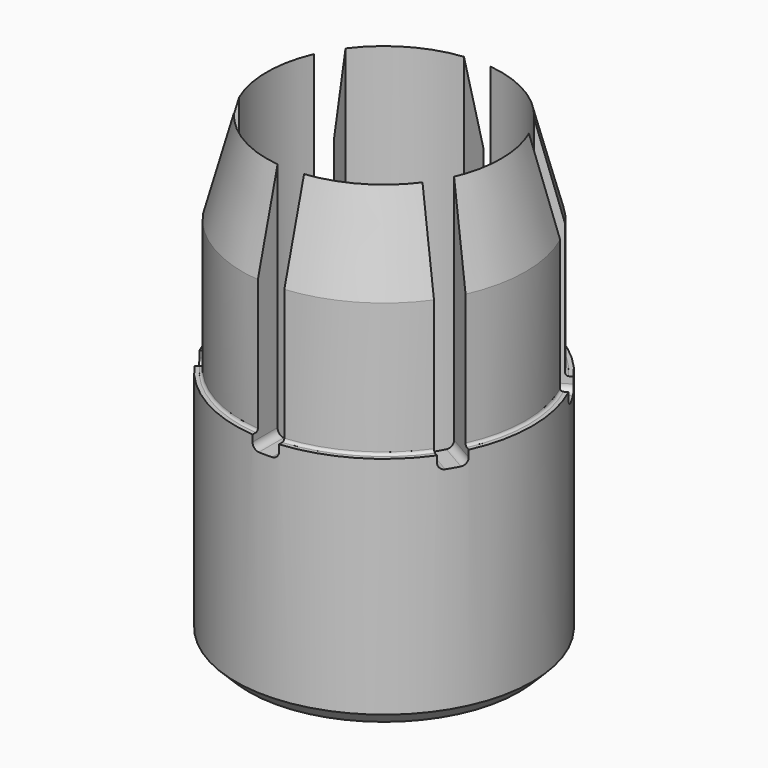
from build123d import *

# Parameters (mm, degrees)
F3_SIZE         = 0.254
F4_W            = 0.508
F4_H            = 3.048
F6_DEPTH        = 4.572
F6_COPIES_COUNT = 6
F7_R            = 0.127
F8_R            = 0.0508


# Not quite as in the source:
# - a pattern or mirror of a feature is missing from the dataset's text; its kind, count and spacing are read off the source's solid


with BuildPart() as f1:
    # F0 (on Front) → F1 (revolve)
    with BuildSketch(Plane.XZ):
        with BuildLine():
            Line((2.2098, 0), (2.8448, 0))
            Line((2.8448, 0), (2.8448, 4.572))
            Line((2.8448, 4.572), (2.7178, 4.572))
            Line((2.7178, 4.572), (2.7178, 7.1363093255))
            Line((2.7178, 7.1363093255), (2.2479, 8.89))
            Line((2.2479, 8.89), (2.2479, 1.397))
            ThreePointArc((2.2479, 1.397), (2.2107025612, 1.3071974388), (2.1209, 1.27))
            Line((2.1209, 1.27), (0, 1.27))
            Line((0, 1.27), (0, 0.3969097134))
            ThreePointArc((0, 0.3969097134), (1.1225811063, 0.2968946462), (2.2098, 0))
        make_face()
    revolve(axis=Axis((0, 0, 7.5646454352), (0, 0, 1)))

    # F3
    f3_edges = [f1.edges().sort_by_distance(p)[0] for p in [
        (-2.8448, 0, 0),
    ]]
    chamfer(f3_edges, length=F3_SIZE)

    # F4 (on offset) → F6 (cut)
    with BuildSketch(Plane.XY.offset(8.89)):
        with Locations((0, 1.524)):
            Rectangle(F4_W, F4_H)
    f6 = extrude(amount=-F6_DEPTH, mode=Mode.SUBTRACT)

    # F6_copies: F6 ×6 about axis
    f6_copies_axis = Axis((0, 0, 0), (0, 0, 1))
    for i in range(1, F6_COPIES_COUNT):
        add(f6.rotate(f6_copies_axis, i * 360 / F6_COPIES_COUNT), mode=Mode.SUBTRACT)

    # F7
    f7_edges = [f1.edges().sort_by_distance(p)[0] for p in [
        (-0.254, 2.533471, 4.318),
        (0.254, 2.533471, 4.318),
        (2.32105, 1.046765, 4.318),
        (2.06705, 1.486706, 4.318),
        (-2.06705, 1.486706, 4.318),
        (-2.32105, 1.046765, 4.318),
        (-2.32105, -1.046765, 4.318),
        (-2.06705, -1.486706, 4.318),
        (-0.254, -2.533471, 4.318),
        (0.254, -2.533471, 4.318),
        (2.06705, -1.486706, 4.318),
        (2.32105, -1.046765, 4.318),
    ]]
    fillet(f7_edges, radius=F7_R)

    # F8
    f8_edges = [f1.edges().sort_by_distance(p)[0] for p in [
        (2.7178, 0, 4.572),
        (1.3589, 2.353684, 4.572),
        (-1.3589, 2.353684, 4.572),
        (1.3589, -2.353684, 4.572),
        (-2.7178, 0, 4.572),
        (-1.3589, -2.353684, 4.572),
    ]]
    fillet(f8_edges, radius=F8_R)


solid = f1.part
